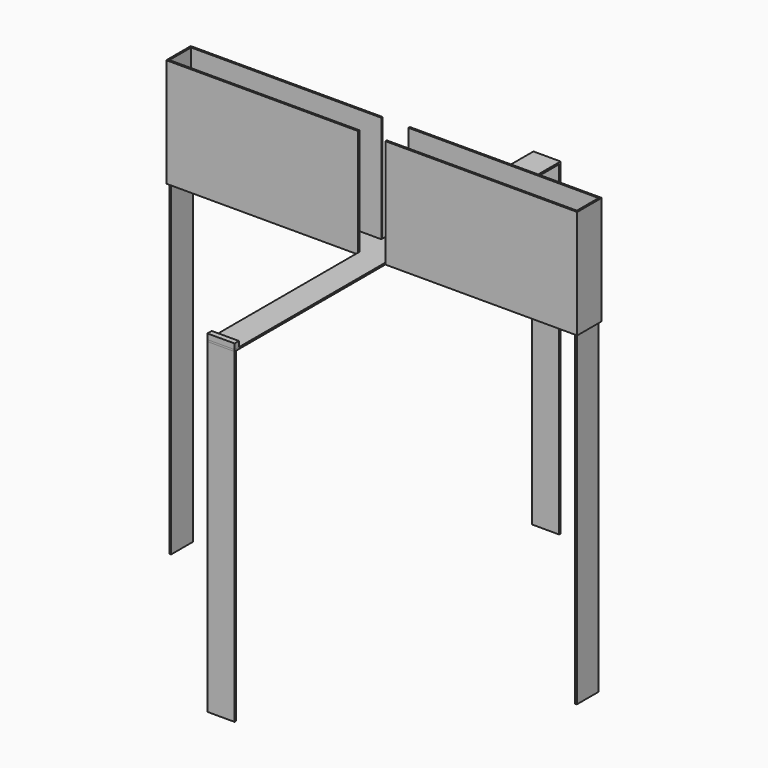
from build123d import *

# Parameters (mm, degrees)
F1_DEPTH = 200
F0_W     = 50
F0_H     = 50
F0_W_2   = 43.65
F0_H_2   = 43.65
F0_H_3   = 6.825
F0_W_3   = 346.825
F0_W_4   = 3.175
F0_H_4   = 3.175
F2_DEPTH = 3.175
F3_W     = 50
F3_H     = 10
F4_DEPTH = 10
F5_DEPTH = 600


# Not quite as in the source:
# - a length typed as a fraction of an inch, garbled in the dataset ("3 / 203.2 mm" for 3/8 in), is restored


with BuildPart() as f1:
    # F0 (on Top) → F1 (new body)
    with BuildSketch(Plane.XY):
        Polygon((-371.825, 25), (-25, 25), (-25, 28.175), (-378.175, 28.175), (-378.175, -28.175), (-25, -28.175), (-25, -25), (-371.825, -25), (-375, -25), (-375, 25), align=None)
    extrude(amount=F1_DEPTH)


with BuildPart() as f1b:
    # F0 (on Top) → F1, piece 2 (new body)
    with BuildSketch(Plane.XY):
        Polygon((371.825, 25), (375, 25), (375, -25), (371.825, -25), (25, -25), (25, -28.175), (378.175, -28.175), (378.175, 28.175), (25, 28.175), (25, 25), align=None)
    extrude(amount=F1_DEPTH)


with BuildPart() as f2:
    # F0 (on Top) → F2 (new body)
    with BuildSketch(Plane.XY):
        Rectangle(F0_W, F0_H)
        Rectangle(F0_W_2, F0_H_2, mode=Mode.SUBTRACT)
        Polygon((25, -28.175), (25, -25), (-25, -25), (-25, -28.175), (-25, -365), (25, -365), align=None)
        with Locations((0, -368.4125)):
            Rectangle(F0_W, F0_H_3)
        with Locations((-198.4125, 0)):
            Rectangle(F0_W_3, F0_H)
        Rectangle(F0_W_2, F0_H_2)
        with Locations((198.4125, 0)):
            Rectangle(F0_W_3, F0_H)
        Polygon((-25, 25), (25, 25), (25, 28.175), (25, 371.825), (-25, 371.825), (-25, 28.175), align=None)
        with Locations((-373.4125, 0)):
            Rectangle(F0_W_4, F0_H)
        with Locations((373.4125, 0)):
            Rectangle(F0_W_4, F0_H)
        with Locations((0, 373.4125)):
            Rectangle(F0_W, F0_H_4)
        with Locations((0, -373.4125)):
            Rectangle(F0_W, F0_H_4)
    extrude(amount=F2_DEPTH)


with BuildPart() as f4:
    # F3 (on face) → F4 (new body)
    with BuildSketch(Plane.XY.offset(3.175)):
        with Locations((0, -370)):
            Rectangle(F3_W, F3_H)
    extrude(amount=F4_DEPTH)


with BuildPart() as f5:
    # F0 (on Top) → F5 (new body)
    with BuildSketch(Plane.XY):
        with Locations((0, 373.4125)):
            Rectangle(F0_W, F0_H_4)
    extrude(amount=-F5_DEPTH)


with BuildPart() as f5b:
    # F0 (on Top) → F5, piece 2 (new body)
    with BuildSketch(Plane.XY):
        with Locations((-373.4125, 0)):
            Rectangle(F0_W_4, F0_H)
    extrude(amount=-F5_DEPTH)


with BuildPart() as f5c:
    # F0 (on Top) → F5, piece 3 (new body)
    with BuildSketch(Plane.XY):
        with Locations((373.4125, 0)):
            Rectangle(F0_W_4, F0_H)
    extrude(amount=-F5_DEPTH)


with BuildPart() as f5d:
    # F0 (on Top) → F5, piece 4 (new body)
    with BuildSketch(Plane.XY):
        with Locations((0, -373.4125)):
            Rectangle(F0_W, F0_H_4)
    extrude(amount=-F5_DEPTH)


solid = Compound([f1.part, f1b.part, f2.part, f4.part, f5.part, f5b.part, f5c.part, f5d.part])
